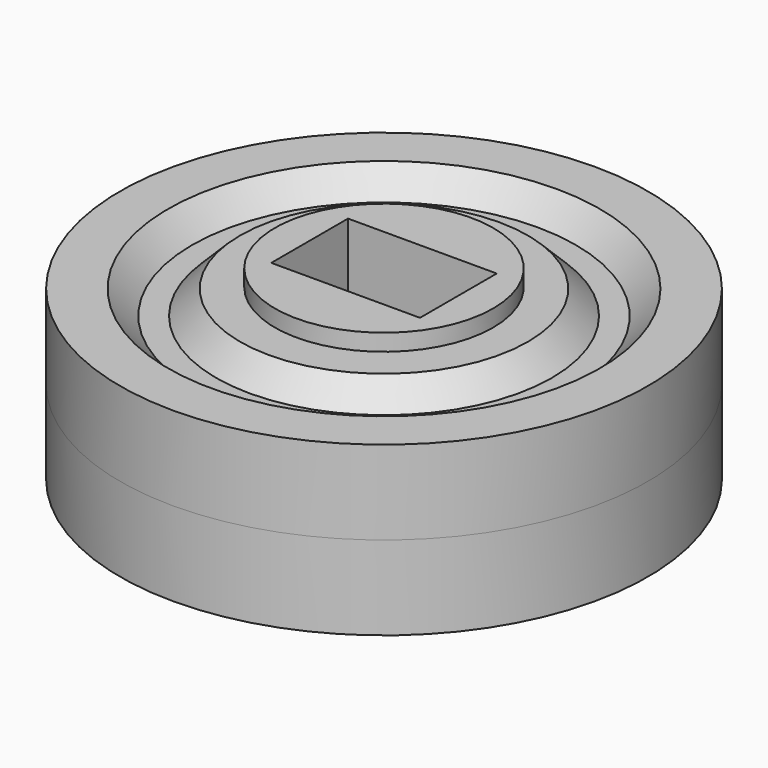
from build123d import *

# Parameters (mm, degrees)
F4_R      = 3.85
F4_W      = 6.2
F4_H      = 4
F9_DEPTH  = 4.25
F11_DEPTH = 5.5
F13_DEPTH = 0.7
F14_R     = 4.55
F14_R_2   = 3.85
F15_DEPTH = 0.7


# Not quite as in the source:
# - a feature of the source that left no trace in its solid (it failed there, or was rolled back) is left out


with BuildPart() as f2:
    # F1 (on Right) → F2 (revolve)
    with BuildSketch(Plane.YZ):
        Polygon((-11, 0), (-4, 0), (-4, 3.5), (-6, 3.5), (-7, 2.5), (-8, 2.5), (-9, 3.5), (-11, 3.5), align=None)
        Polygon((8, 2.5), (7, 2.5), (6, 3.5), (4, 3.5), (4, 0), (11, 0), (11, 3.5), (9, 3.5), align=None)
    revolve(axis=Axis((0, 0, 2.2127844859), (0, 0, 1)))


with BuildPart() as f3_1:
    # F3: instance of F2
    add(f2.part.mirror(Plane.XY))


with BuildPart() as f2_1:
    add(f2.part)

    # F8: F2 across plane
    add(f2.part.mirror(Plane.XY))


with BuildPart() as f9:
    # F4 (on Top) → F9 (new body, symmetric)
    with BuildSketch(Plane.XY):
        Circle(F4_R)
        Rectangle(F4_W, F4_H, mode=Mode.SUBTRACT)
    extrude(amount=F9_DEPTH, both=True)

    # F10 (on face) → F11 (cut)
    with BuildSketch(Plane(origin=(0, 0, -4.25), x_dir=(1, 0, 0), z_dir=(0, 0, -1))):
        with BuildLine():
            Line((-3.1, -2), (-3.1, 2))
            Line((-3.1, 2), (-3.2897568299, 2))
            ThreePointArc((-3.2897568299, 2), (-3.85, 0), (-3.2897568299, -2))
            Line((-3.2897568299, -2), (-3.1, -2))
        make_face()
        with BuildLine():
            Line((3.2897568299, 2), (3.1, 2))
            Line((3.1, 2), (3.1, -2))
            Line((3.1, -2), (3.2897568299, -2))
            ThreePointArc((3.2897568299, -2), (3.7072944174, -1.0384931884), (3.85, 0))
            ThreePointArc((3.85, 0), (3.7072944174, 1.0384931884), (3.2897568299, 2))
        make_face()
    extrude(amount=-F11_DEPTH, mode=Mode.SUBTRACT)

    # F12 (on face) → F13 (join)
    with BuildSketch(Plane(origin=(0, 0, -4.25), x_dir=(1, 0, 0), z_dir=(0, 0, -1))):
        with BuildLine():
            Line((-3.2897568299, -2), (-4.0868692174, -2))
            ThreePointArc((-4.0868692174, -2), (0, -4.55), (4.0868692174, -2))
            Line((4.0868692174, -2), (3.2897568299, -2))
            ThreePointArc((3.2897568299, -2), (0, -3.85), (-3.2897568299, -2))
        make_face()
        with BuildLine():
            ThreePointArc((4.0868692174, 2), (0, 4.55), (-4.0868692174, 2))
            Line((-4.0868692174, 2), (-3.2897568299, 2))
            ThreePointArc((-3.2897568299, 2), (0, 3.85), (3.2897568299, 2))
            Line((3.2897568299, 2), (4.0868692174, 2))
        make_face()
    extrude(amount=-F13_DEPTH)

    # F14 (on face) → F15 (join)
    with BuildSketch(Plane.XY.offset(4.25)):
        Circle(F14_R)
        Circle(F14_R_2, mode=Mode.SUBTRACT)
    extrude(amount=-F15_DEPTH)


solid = Compound([f2_1.part, f9.part])
